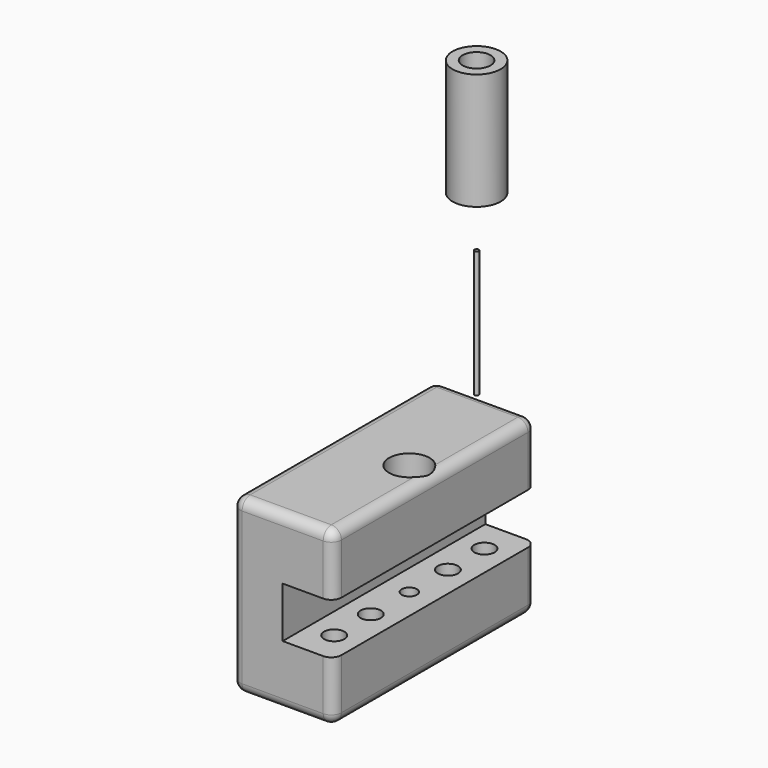
from build123d import *

# Parameters (mm, degrees)
F1_DEPTH     = 50
F3_D         = 8
F3_DEPTH     = 12
F3_TIP       = 2.4034424761
F5_D         = 3
F7_D         = 4
F7_DEPTH     = 12.001
F9_D         = 4
F9_DEPTH     = 12.001
F11_D        = 4
F11_DEPTH    = 12.001
F13_D        = 4
F13_DEPTH    = 12.001
F14_T1_DEPTH = 60
F15_R        = 2
F16_R        = 2
F17_R        = 2
F20_R        = 0.430653221
F21_DEPTH    = 25


# Not quite as in the source:
# - a fillet or chamfer that OpenCascade refuses, or shapes differently, is made with other operations: its cross-section is extruded or revolved along the edge and cut away or added


with BuildPart() as f1:
    # F0 (on Front) → F1 (new body)
    with BuildSketch(Plane.XZ):
        Polygon((21.6415318622, 12), (1.6415318622, 12), (1.6415318622, -22), (21.6415318622, -22), (21.6415318622, -10), (11.6415318622, -10), (11.6415318622, 0), (21.6415318622, 0), align=None)
    extrude(amount=F1_DEPTH)

    # F3
    with Locations(Plane.XY.offset(12)):
        with Locations((16.6415318622, -25)):
            Hole(F3_D / 2, depth=F3_DEPTH)
            with Locations((0, 0, -(F3_DEPTH + F3_TIP / 2))):  # 118° drill point
                Cone(0, F3_D / 2, F3_TIP, mode=Mode.SUBTRACT)

    # F5 (through all)
    with Locations(Plane.XY.offset(-10)):
        with Locations((16.6415318622, -25)):
            Hole(F5_D / 2)

    # F7 (through all, one way)
    with BuildSketch(Plane.XY.offset(-10)):
        with Locations((16.6415318622, -34.52)):
            Circle(F7_D / 2)
    extrude(amount=-F7_DEPTH, mode=Mode.SUBTRACT)

    # F9 (through all, one way)
    with BuildSketch(Plane.XY.offset(-10)):
        with Locations((16.6415318622, -15.48)):
            Circle(F9_D / 2)
    extrude(amount=-F9_DEPTH, mode=Mode.SUBTRACT)

    # F11 (through all, one way)
    with BuildSketch(Plane.XY.offset(-10)):
        with Locations((16.6415318622, -6.46)):
            Circle(F11_D / 2)
    extrude(amount=-F11_DEPTH, mode=Mode.SUBTRACT)

    # F13 (through all, one way)
    with BuildSketch(Plane.XY.offset(-10)):
        with Locations((16.6415318622, -43.54)):
            Circle(F13_D / 2)
    extrude(amount=-F13_DEPTH, mode=Mode.SUBTRACT)

    # F14: fillet of radius 2 on 1 edges, made by hand

    # F14_s2 → F14_t1 (cut)
    with BuildSketch(Plane.XZ.offset(-5)):
        with BuildLine():
            ThreePointArc((21.6415318622, 10), (21.0557454246, 11.4142135624), (19.6415318622, 12))
            Line((19.6415318622, 12), (21.6415318622, 12))
            Line((21.6415318622, 12), (21.6415318622, 10))
        make_face()
    extrude(amount=F14_T1_DEPTH, mode=Mode.SUBTRACT)

    # F15
    f15_edges = [f1.edges().sort_by_distance(p)[0] for p in [
        (21.641532, -25, -22),
    ]]
    fillet(f15_edges, radius=F15_R)

    # F16
    f16_edges = [f1.edges().sort_by_distance(p)[0] for p in [
        (1.641532, -25, 12),
        (1.641532, -25, -22),
    ]]
    fillet(f16_edges, radius=F16_R)

    # F17
    f17_edges = [f1.edges().sort_by_distance(p)[0] for p in [
        (11.641532, -50, -22),
        (1.641532, -50, -5),
        (11.641532, -50, 12),
        (11.641532, 0, 12),
        (1.641532, 0, -5),
        (11.641532, 0, -22),
        (2.227318, 0, -21.414214),
        (21.055745, 0, -21.414214),
        (21.641532, 0, -15),
        (2.227318, 0, 11.414214),
        (21.055745, 0, 11.414214),
        (21.641532, 0, 5),
        (2.227318, -50, -21.414214),
        (21.055745, -50, -21.414214),
        (21.641532, -50, -15),
        (2.227318, -50, 11.414214),
        (21.055745, -50, 11.414214),
        (21.641532, -50, 5),
    ]]
    fillet(f17_edges, radius=F17_R)


with BuildPart() as f21:
    # F20 (on face) → F21 (new body)
    with BuildSketch(Plane.XY.offset(12)):
        with Locations((9.9141315413, 0)):
            Circle(F20_R)
    extrude(amount=F21_DEPTH)


with BuildPart() as f22:
    # F18 (on Front) → F22 (revolve)
    with BuildSketch(Plane.XZ):
        Polygon((11.1641315413, 47.0304564509), (14.6641315413, 47.0304564509), (14.6641315413, 70.0304564509), (12.6641315413, 70.0304564509), (12.6641315413, 50.0304564509), (11.1641315413, 50.0304564509), align=None)
    revolve(axis=Axis((9.9141315413, 0, 12), (0, 0, -1)))


solid = Compound([f1.part, f21.part, f22.part])
